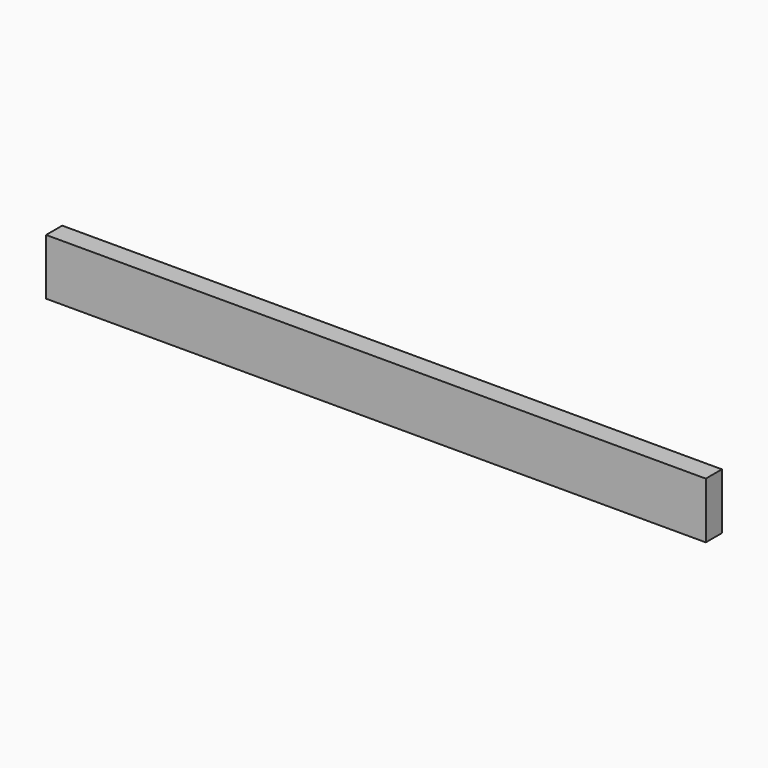
from build123d import *

# Parameters (mm, degrees)
F0_W     = 596.9
F0_H     = 50.8
F1_DEPTH = 18.25625


# Not quite as in the source:
# - a length typed as a fraction of an inch, garbled in the dataset ("3 / 203.2 mm" for 3/8 in), is restored


with BuildPart() as f1:
    # F0 (on Front) → F1 (new body)
    with BuildSketch(Plane.XZ):
        with Locations((181.2523299575, 2.6312100977)):
            Rectangle(F0_W, F0_H)
    extrude(amount=F1_DEPTH)


solid = f1.part
